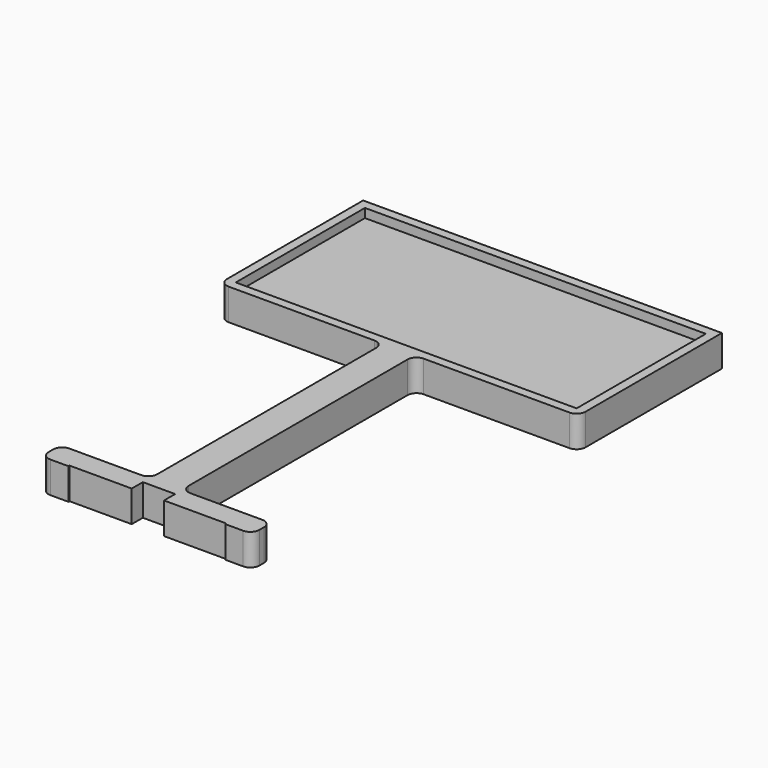
from build123d import *

# Parameters (mm, degrees)
F0_W     = 6
F0_H     = 0.3
F1_DEPTH = 7
F2_W     = 76
F2_H     = 36
F3_DEPTH = 2
F4_R     = 2


# Not quite as in the source:
# - a feature names something its author has since deleted; it is built from what else it names


with BuildPart() as f1:
    # F0 (on Top) → F1 (new body)
    with BuildSketch(Plane.XY):
        Polygon((3.5, 0), (-3.5, 0), (-3.5, -65), (-23.5, -65), (-23.5, -70), (-17.5, -70), (-3.6, -70), (-3.6, -66.9), (3.6, -66.9), (3.6, -70), (17.5, -70), (23.5, -70), (23.5, -65), (3.5, -65), align=None)
        with Locations((-20.5, -70.15)):
            Rectangle(F0_W, F0_H)
        with Locations((20.5, -70.15)):
            Rectangle(F0_W, F0_H)
        Polygon((-40, 40), (-40, 0), (-3.5, 0), (3.5, 0), (40, 0), (40, 40), align=None)
    extrude(amount=F1_DEPTH)

    # F2 (on face) → F3 (cut)
    with BuildSketch(Plane.XY.offset(7)):
        with Locations((0, 20)):
            Rectangle(F2_W, F2_H)
    extrude(amount=-F3_DEPTH, mode=Mode.SUBTRACT)

    # F4
    f4_edges = [f1.edges().sort_by_distance(p)[0] for p in [
        (-3.5, 0, 3.5),
        (3.5, 0, 3.5),
        (3.5, -65, 3.5),
        (-3.5, -65, 3.5),
        (-23.5, -65, 3.5),
        (23.5, -65, 3.5),
        (-23.5, -70.3, 3.5),
        (23.5, -70.3, 3.5),
        (40, 0, 3.5),
        (-40, 0, 3.5),
    ]]
    fillet(f4_edges, radius=F4_R)


solid = f1.part
